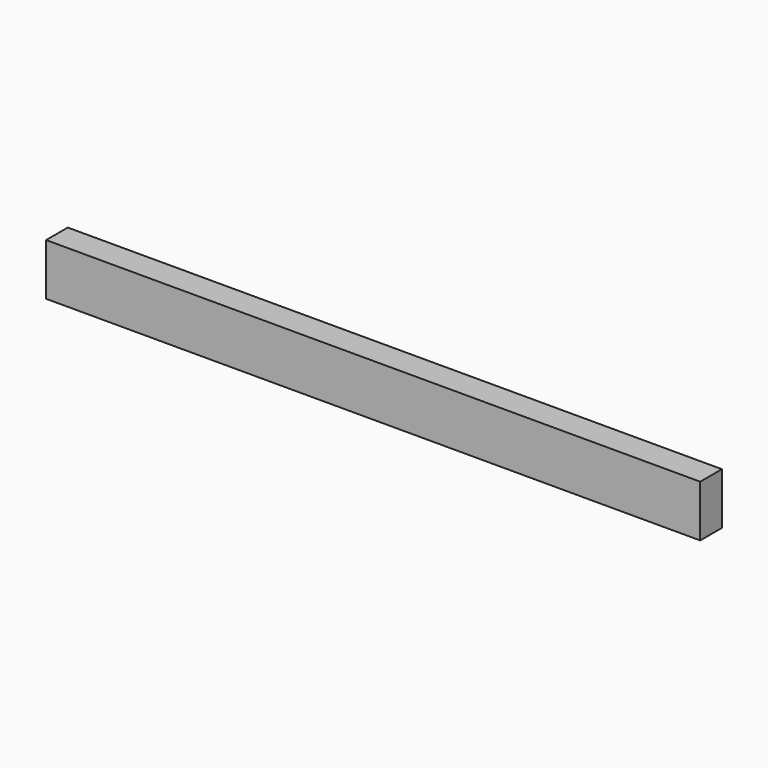
from build123d import *

# Parameters (mm, degrees)
F0_W     = 34.925
F0_H     = 66.675
F1_DEPTH = 421.48125


# Not quite as in the source:
# - a length typed as a fraction of an inch, garbled in the dataset ("3 / 203.2 mm" for 3/8 in), is restored


with BuildPart() as f1:
    # F0 (on Right) → F1 (new body, symmetric)
    with BuildSketch(Plane.YZ):
        with Locations((17.4625, 33.3375)):
            Rectangle(F0_W, F0_H)
    extrude(amount=F1_DEPTH, both=True)


solid = f1.part
